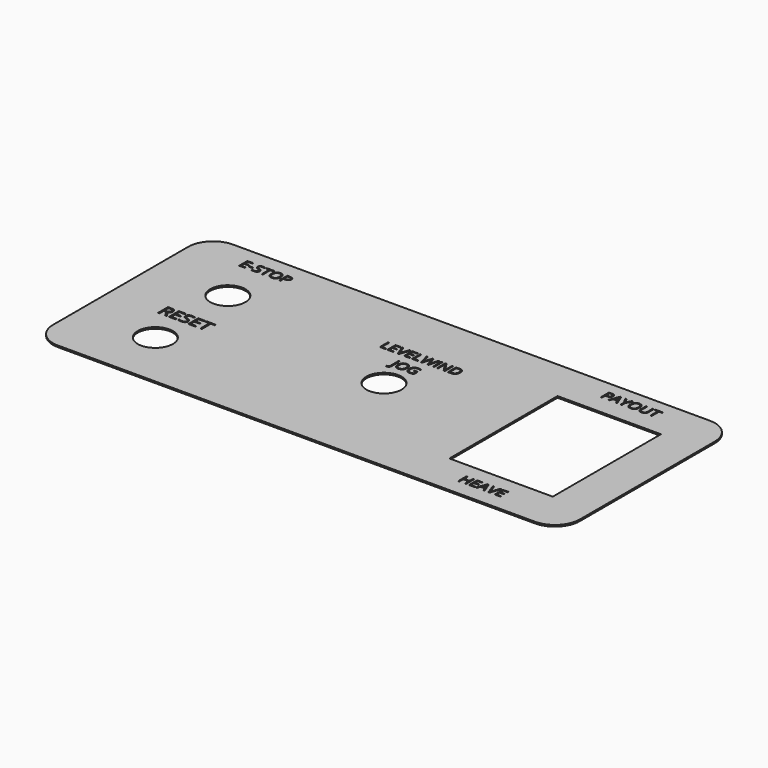
from build123d import *

# Parameters (mm, degrees)
F0_W           = 336.55
F0_H           = 139.7
F0_R           = 11.25
F0_W_2         = 66.04
F0_H_2         = 86.36
F1_DEPTH       = 1
F2_R           = 15.88
F3_TEXT_SIZE   = 9.2297792435
F3_TEXT_SIZE_2 = 11.1980798576
F4_DEPTH       = 0.9


# Not quite as in the source:
# - Text() gives the source's letters only with a copy of the font that has no kerning and outlines rounded to 1/6400 em; it was checked with that copy


with BuildPart() as f1:
    # F0 (on Top) → F1 (new body)
    with BuildSketch(Plane.XY):
        with Locations((168.275, 69.85)):
            Rectangle(F0_W, F0_H)
        with Locations((48.39, 37.08)):
            Circle(F0_R, mode=Mode.SUBTRACT)
        with Locations((48.39, 95)):
            Circle(F0_R, mode=Mode.SUBTRACT)
        with Locations((168.275, 69.85)):
            Circle(F0_R, mode=Mode.SUBTRACT)
        with Locations((277.62, 69.85)):
            Rectangle(F0_W_2, F0_H_2, mode=Mode.SUBTRACT)
    extrude(amount=F1_DEPTH)

    # F2
    f2_edges = [f1.edges().sort_by_distance(p)[0] for p in [
        (0, 0, 0.5),
        (336.55, 0, 0.5),
        (336.55, 139.7, 0.5),
        (0, 139.7, 0.5),
    ]]
    fillet(f2_edges, radius=F2_R)

    # F3 (on face) → F4 (cut)
    with BuildSketch(Plane.XY.offset(1)):
        with Locations((31.7237582058, 123.7413287163)):
            Text('E-STOP', F3_TEXT_SIZE, font='Open Sans', text_align=(TextAlign.LEFT, TextAlign.BOTTOM))
        with Locations((31.7237582058, 58.7049633098)):
            Text('RESET', F3_TEXT_SIZE_2, font='Open Sans', text_align=(TextAlign.LEFT, TextAlign.BOTTOM))
        with Locations((141.3753610104, 99.0139916539)):
            Text('LEVELWIND', F3_TEXT_SIZE, font='Open Sans', text_align=(TextAlign.LEFT, TextAlign.BOTTOM))
        with Locations((158.1634641625, 86.4614918828)):
            Text('JOG', F3_TEXT_SIZE, font='Open Sans', text_align=(TextAlign.LEFT, TextAlign.BOTTOM))
        with Locations((261.3346483558, 125.4742369056)):
            Text('PAYOUT', F3_TEXT_SIZE, font='Open Sans', text_align=(TextAlign.LEFT, TextAlign.BOTTOM))
        with Locations((262.3953130096, 10.3503847495)):
            Text('HEAVE', F3_TEXT_SIZE, font='Open Sans', text_align=(TextAlign.LEFT, TextAlign.BOTTOM))
    extrude(amount=-F4_DEPTH, mode=Mode.SUBTRACT)


solid = f1.part
